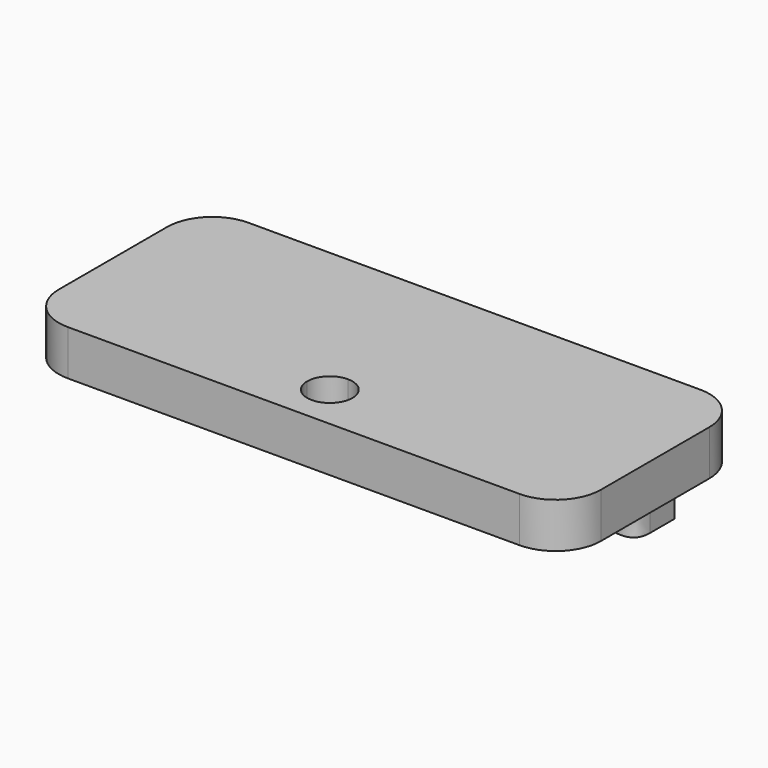
from build123d import *

# Parameters (mm, degrees)
F1_DEPTH     = 5.08
F2_TEXT_SIZE = 9.8660732349
F3_DEPTH     = 2.54


# Not quite as in the source:
# - Text() gives the source's letters only with a copy of the font that has no kerning and outlines rounded to 1/6400 em; it was checked with that copy


with BuildPart() as f1:
    # F0 (on Top) → F1 (new body)
    with BuildSketch(Plane.XY):
        with BuildLine():
            Line((-25.4, 0), (-25.4, 2.54))
            ThreePointArc((-25.4, 2.54), (-28.9921024484, 4.0278975516), (-30.48, 7.62))
            Line((-30.48, 7.62), (-30.48, -7.62))
            ThreePointArc((-30.48, -7.62), (-28.9921024484, -4.0278975516), (-25.4, -2.54))
            Line((-25.4, -2.54), (-25.4, 0))
        make_face()
        with BuildLine():
            Line((-20.32, -7.62), (-25.4, -7.62))
            Line((-25.4, -7.62), (-28.4995739001, -11.6448033042))
            ThreePointArc((-28.4995739001, -11.6448033042), (-27.037131518, -12.4289708247), (-25.4, -12.7))
            ThreePointArc((-25.4, -12.7), (-21.8078975516, -11.2121024484), (-20.32, -7.62))
        make_face()
        with BuildLine():
            Line((-25.4, -7.62), (-25.4, -2.54))
            ThreePointArc((-25.4, -2.54), (-28.9921024484, -4.0278975516), (-30.48, -7.62))
            ThreePointArc((-30.48, -7.62), (-29.9580826787, -9.8628290826), (-28.4995739001, -11.6448033042))
            Line((-28.4995739001, -11.6448033042), (-25.4, -7.62))
        make_face()
        with BuildLine():
            ThreePointArc((-20.32, -7.62), (-21.8078975516, -4.0278975516), (-25.4, -2.54))
            Line((-25.4, -2.54), (-25.4, -7.62))
            Line((-25.4, -7.62), (-20.32, -7.62))
        make_face()
        with BuildLine():
            Line((-20.32, 7.62), (-25.4, 7.62))
            Line((-25.4, 7.62), (-25.4, 2.54))
            ThreePointArc((-25.4, 2.54), (-21.8078975516, 4.0278975516), (-20.32, 7.62))
        make_face()
        with BuildLine():
            Line((-25.4, 2.54), (-25.4, 7.62))
            Line((-25.4, 7.62), (-20.32, 7.62))
            ThreePointArc((-20.32, 7.62), (-21.8078975516, 11.2121024484), (-25.4, 12.7))
            ThreePointArc((-25.4, 12.7), (-28.9921024484, 11.2121024484), (-30.48, 7.62))
            ThreePointArc((-30.48, 7.62), (-28.9921024484, 4.0278975516), (-25.4, 2.54))
        make_face()
        with BuildLine():
            ThreePointArc((-25.4, 12.7), (-21.8078975516, 11.2121024484), (-20.32, 7.62))
            Line((-20.32, 7.62), (20.32, 7.62))
            ThreePointArc((20.32, 7.62), (21.8078975516, 11.2121024484), (25.4, 12.7))
            Line((25.4, 12.7), (-25.4, 12.7))
        make_face()
        with BuildLine():
            ThreePointArc((25.4, 12.7), (21.8078975516, 11.2121024484), (20.32, 7.62))
            Line((20.32, 7.62), (25.4, 7.62))
            Line((25.4, 7.62), (25.4, 2.54))
            ThreePointArc((25.4, 2.54), (28.9921024484, 4.0278975516), (30.48, 7.62))
            ThreePointArc((30.48, 7.62), (28.9921024484, 11.2121024484), (25.4, 12.7))
        make_face()
        with BuildLine():
            ThreePointArc((30.48, 7.62), (28.9921024484, 4.0278975516), (25.4, 2.54))
            Line((25.4, 2.54), (25.4, -2.54))
            ThreePointArc((25.4, -2.54), (28.9921024484, -4.0278975516), (30.48, -7.62))
            Line((30.48, -7.62), (30.48, 7.62))
        make_face()
        with BuildLine():
            Line((25.4, 7.62), (20.32, 7.62))
            ThreePointArc((20.32, 7.62), (21.8078975516, 4.0278975516), (25.4, 2.54))
            Line((25.4, 2.54), (25.4, 7.62))
        make_face()
        with BuildLine():
            ThreePointArc((30.48, -7.62), (28.9921024484, -4.0278975516), (25.4, -2.54))
            Line((25.4, -2.54), (25.4, -7.62))
            Line((25.4, -7.62), (20.32, -7.62))
            ThreePointArc((20.32, -7.62), (21.8078975516, -11.2121024484), (25.4, -12.7))
            ThreePointArc((25.4, -12.7), (28.9921024484, -11.2121024484), (30.48, -7.62))
        make_face()
        with BuildLine():
            Line((25.4, -7.62), (25.4, -2.54))
            ThreePointArc((25.4, -2.54), (21.8078975516, -4.0278975516), (20.32, -7.62))
            Line((20.32, -7.62), (25.4, -7.62))
        make_face()
        with BuildLine():
            Line((-2.54, -7.62), (-20.32, -7.62))
            ThreePointArc((-20.32, -7.62), (-21.8078975516, -11.2121024484), (-25.4, -12.7))
            Line((-25.4, -12.7), (0, -12.7))
            Line((0, -12.7), (0, -10.16))
            ThreePointArc((0, -10.16), (-1.107287049, -9.9059386236), (-1.9930631755, -9.1945790481))
            ThreePointArc((-1.9930631755, -9.1945790481), (-2.3993728832, -8.4534325211), (-2.54, -7.62))
        make_face()
        with BuildLine():
            ThreePointArc((25.4, -12.7), (21.8078975516, -11.2121024484), (20.32, -7.62))
            Line((20.32, -7.62), (2.54, -7.62))
            ThreePointArc((2.54, -7.62), (1.7960512242, -9.4160512242), (0, -10.16))
            Line((0, -10.16), (0, -12.7))
            Line((0, -12.7), (25.4, -12.7))
        make_face()
        with BuildLine():
            Line((0, 0), (-25.4, 0))
            Line((-25.4, 0), (-25.4, -2.54))
            ThreePointArc((-25.4, -2.54), (-21.8078975516, -4.0278975516), (-20.32, -7.62))
            Line((-20.32, -7.62), (-2.54, -7.62))
            ThreePointArc((-2.54, -7.62), (-1.7960512242, -5.8239487758), (0, -5.08))
            Line((0, -5.08), (0, 0))
        make_face()
        with BuildLine():
            Line((20.32, 7.62), (-20.32, 7.62))
            ThreePointArc((-20.32, 7.62), (-21.8078975516, 4.0278975516), (-25.4, 2.54))
            Line((-25.4, 2.54), (-25.4, 0))
            Line((-25.4, 0), (0, 0))
            Line((0, 0), (0, -5.08))
            ThreePointArc((0, -5.08), (1.7960512242, -5.8239487758), (2.54, -7.62))
            Line((2.54, -7.62), (20.32, -7.62))
            ThreePointArc((20.32, -7.62), (21.8078975516, -4.0278975516), (25.4, -2.54))
            Line((25.4, -2.54), (25.4, 2.54))
            ThreePointArc((25.4, 2.54), (21.8078975516, 4.0278975516), (20.32, 7.62))
        make_face()
    extrude(amount=F1_DEPTH)

    # F2 (on face) → F3 (join)
    with BuildSketch(Plane(origin=(0, 0, 0), x_dir=(1, 0, 0), z_dir=(0, 0, -1))):
        with Locations((-30.48, -3.5517863646)):
            Text('Lorem Ipsum', F2_TEXT_SIZE, font='Open Sans', text_align=(TextAlign.LEFT, TextAlign.BOTTOM))
    extrude(amount=F3_DEPTH)


solid = f1.part
